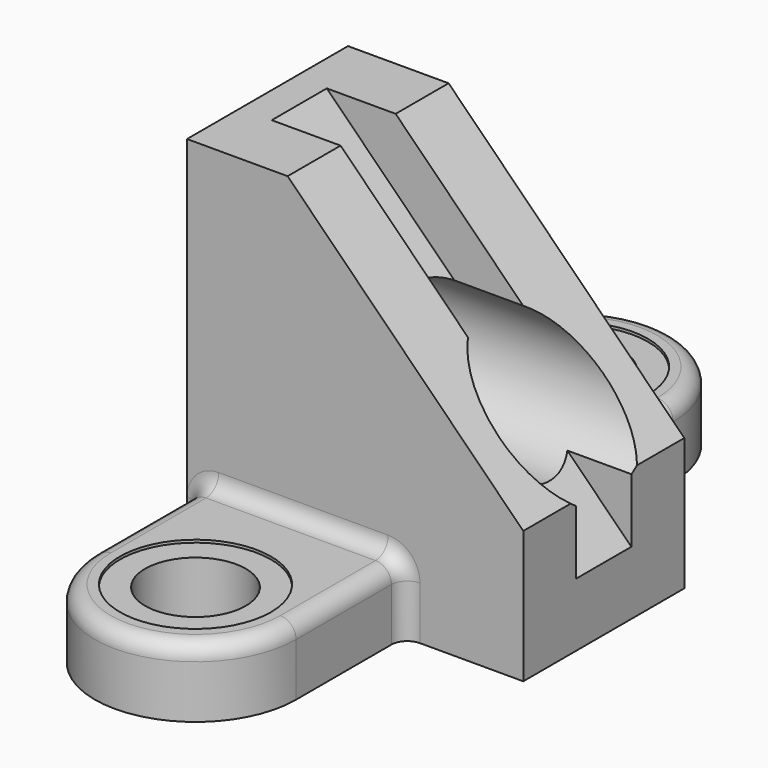
from build123d import *

# Parameters (mm, degrees)
F1_DEPTH  = 38
F3_DEPTH  = 13
F5_DEPTH  = 26
F6_R      = 19
F7_DEPTH  = 26.001
F6_R_2    = 28.5
F8_DEPTH  = 1
F9_R      = 5.99999
F11_R     = 25
F12_DEPTH = 127.001


# Not quite as in the source:
# - a fillet or chamfer is up to 0.001 mm smaller than in the source, because OpenCascade refuses the exact size


with BuildPart() as f1:
    # F0 (on Front) → F1 (new body)
    with BuildSketch(Plane.XZ):
        Polygon((-60.1392750332, 139), (-60.1392750332, 0), (66.8607249668, 0), (66.8607249668, 50), (-22.1392750332, 139), align=None)
    extrude(amount=F1_DEPTH)

    # F2 (on face) → F3 (cut)
    with BuildSketch(Plane(origin=(0, 0, 0), x_dir=(-1, 0, 0), z_dir=(0, 1, 0))):
        Polygon((-66.8607249668, 24), (48.1392750332, 139), (22.1392750332, 139), (-66.8607249668, 50), align=None)
    extrude(amount=-F3_DEPTH, mode=Mode.SUBTRACT)

    # F4 (on Top) → F5 (join)
    with BuildSketch(Plane.XY):
        with BuildLine():
            Line((21.8607249668, -38), (-54.1392750332, -38))
            Line((-54.1392750332, -38), (-54.1392750332, -89))
            ThreePointArc((-54.1392750332, -89), (-16.1392750332, -127), (21.8607249668, -89))
            Line((21.8607249668, -89), (21.8607249668, -38))
        make_face()
    extrude(amount=F5_DEPTH)

    # F6 (on face) → F7 (cut, through all)
    with BuildSketch(Plane.XY.offset(26)):
        with Locations((-16.1392750332, -89)):
            Circle(F6_R)
    extrude(amount=-F7_DEPTH, mode=Mode.SUBTRACT)

    # F6 (on face) → F8 (cut)
    with BuildSketch(Plane.XY.offset(26)):
        with Locations((-16.1392750332, -89)):
            Circle(F6_R_2)
        with Locations((-16.1392750332, -89)):
            Circle(F6_R, mode=Mode.SUBTRACT)
    extrude(amount=-F8_DEPTH, mode=Mode.SUBTRACT)

    # F9 (radius 6 in the source; OpenCascade refuses exactly that, so slightly less here)
    f9_edges = [f1.edges().sort_by_distance(p)[0] for p in [
        (-16.139275, -38, 26),
        (21.860725, -38, 13),
        (-54.139275, -38, 13),
        (-54.139275, -63.5, 26),
    ]]
    fillet(f9_edges, radius=F9_R)

    # F10: F1 across plane


with BuildPart() as f1_1:
    add(f1.part)
    add(f1.part.mirror(Plane.XZ))

    # F11 (on face) → F12 (cut, through all)
    with BuildSketch(Plane(origin=(-60.1392750332, 0, 0), x_dir=(0, -1, 0), z_dir=(-1, 0, 0))):
        with Locations((0, 69.5)):
            Circle(F11_R)
    extrude(amount=-F12_DEPTH, mode=Mode.SUBTRACT)


solid = f1_1.part
